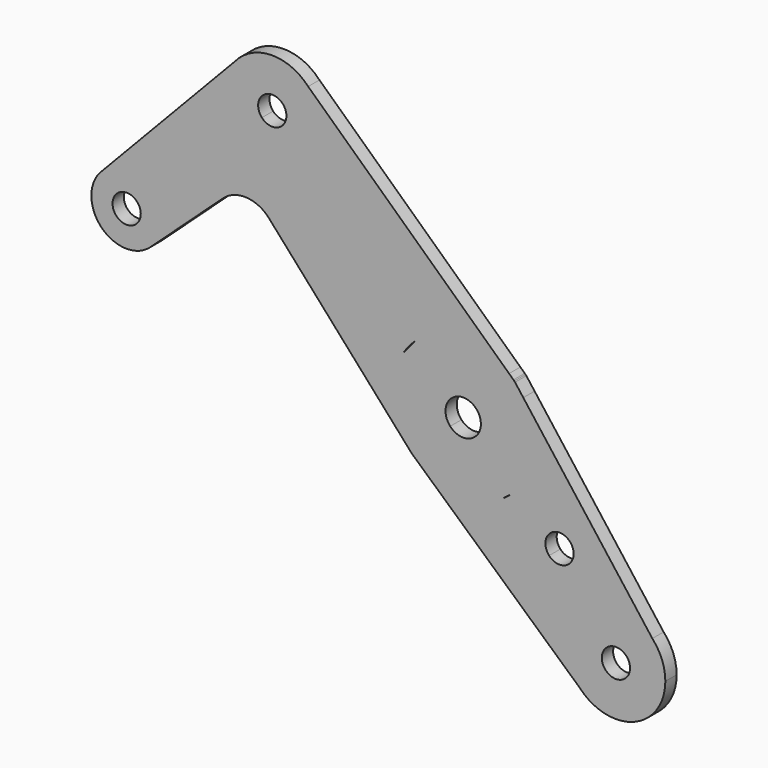
from build123d import *

# Parameters (mm, degrees)
F1_DEPTH = 3.175


with BuildPart() as f1:
    # F0 (on Front) → F1 (new body)
    with BuildSketch(Plane.XZ):
        with BuildLine():
            ThreePointArc((-2.6877932952, 2.9286835289), (1.5995582019, 3.6390704265), (3.9751, 0))
            ThreePointArc((3.9751, 0), (3.6390704265, -1.5995582019), (2.6877932952, -2.9286835289))
            Line((2.6877932952, -2.9286835289), (10.7339987827, -11.6960204828))
            ThreePointArc((10.7339987827, -11.6960204828), (14.5330288597, -6.3880119883), (15.875, 0))
            ThreePointArc((15.875, 0), (15.2734304328, 4.3287351287), (13.5143136611, 8.3294028158))
            Line((13.5143136611, 8.3294028158), (11.6590601378, 10.7741329908))
            Line((11.6590601378, 10.7741329908), (11.4851871667, 10.9592928944))
            Line((11.4851871667, 10.9592928944), (11.3083739877, 11.1416472191))
            Line((11.3083739877, 11.1416472191), (10.3225973322, 12.0606637179))
            ThreePointArc((10.3225973322, 12.0606637179), (-0.2748708071, 15.8726201693), (-10.7339987827, 11.6960204828))
            Line((-10.7339987827, 11.6960204828), (-2.6877932952, 2.9286835289))
        make_face()
        with BuildLine():
            ThreePointArc((-2.9286835289, -2.6877932952), (-3.9714488487, 0.1703351178), (-2.6877932952, 2.9286835289))
            Line((-2.6877932952, 2.9286835289), (-10.7339987827, 11.6960204828))
            Line((-10.7339987827, 11.6960204828), (-13.3268527784, 8.6261590538))
            ThreePointArc((-13.3268527784, 8.6261590538), (-15.8291292061, -1.2059409505), (-11.8662618768, -10.5454944915))
            Line((-11.8662618768, -10.5454944915), (-11.6960204828, -10.7339987827))
            Line((-11.6960204828, -10.7339987827), (-2.9286835289, -2.6877932952))
        make_face()
        with BuildLine():
            Line((10.7339987827, -11.6960204828), (2.6877932952, -2.9286835289))
            ThreePointArc((2.6877932952, -2.9286835289), (-0.1703351178, -3.9714488487), (-2.9286835289, -2.6877932952))
            Line((-2.9286835289, -2.6877932952), (-11.6960204828, -10.7339987827))
            Line((-11.6960204828, -10.7339987827), (-11.5227849075, -10.9197551701))
            Line((-11.5227849075, -10.9197551701), (-9.6887004006, -12.5755600093))
            ThreePointArc((-9.6887004006, -12.5755600093), (-0.5030588817, -15.8670273448), (8.8726348179, -13.1640410357))
            Line((8.8726348179, -13.1640410357), (10.7339987827, -11.6960204828))
        make_face()
        with BuildLine():
            Line((-35.5304524208, 38.714826384), (-10.7339987827, 11.6960204828))
            ThreePointArc((-10.7339987827, 11.6960204828), (-0.2748708071, 15.8726201693), (10.3225973322, 12.0606637179))
            Line((10.3225973322, 12.0606637179), (-34.8667395835, 54.189624641))
            ThreePointArc((-34.8667395835, 54.189624641), (-32.7298053677, 50.7575739011), (-31.9836005106, 46.7840819312))
            ThreePointArc((-31.9836005106, 46.7840819312), (-32.9094460222, 42.3768990566), (-35.5304524208, 38.714826384))
        make_face()
        with BuildLine():
            ThreePointArc((-13.3268527784, 8.6261590538), (-12.1279494046, 10.2434597788), (-10.7339987827, 11.6960204828))
            Line((-10.7339987827, 11.6960204828), (-35.5304524208, 38.714826384))
            ThreePointArc((-35.5304524208, 38.714826384), (-43.4053109787, 35.8417471462), (-51.0052506778, 39.3785392213))
            Line((-51.0052506778, 39.3785392213), (-69.8368422411, 22.0958847311))
            ThreePointArc((-69.8368422411, 22.0958847311), (-68.2881475559, 19.6085836711), (-67.7473524824, 16.7288853397))
            ThreePointArc((-67.7473524824, 16.7288853397), (-68.4183380526, 13.5348793456), (-70.3178530911, 10.8808750983))
            Line((-70.3178530911, 10.8808750983), (-54.0081981098, 25.8490274689))
            ThreePointArc((-54.0081981098, 25.8490274689), (-48.7323738618, 27.7047005709), (-43.6967288942, 25.2715700939))
            Line((-43.6967288942, 25.2715700939), (-20.9173687453, -0.3607843802))
            Line((-20.9173687453, -0.3607843802), (-13.3268527784, 8.6261590538))
        make_face()
        with BuildLine():
            Line((19.3211978133, -21.0528368739), (10.7339987827, -11.6960204828))
            ThreePointArc((10.7339987827, -11.6960204828), (9.830757416, -12.4648238507), (8.8726348179, -13.1640410357))
            Line((8.8726348179, -13.1640410357), (-0.6862483149, -20.7029410933))
            Line((-0.6862483149, -20.7029410933), (26.1615817665, -44.9410646928))
            ThreePointArc((26.1615817665, -44.9410646928), (23.2465029972, -36.9510890975), (26.8349969566, -29.240051207))
            Line((26.8349969566, -29.240051207), (19.3211978133, -21.0528368739))
        make_face()
        with BuildLine():
            ThreePointArc((15.875, 0), (14.5330288597, -6.3880119883), (10.7339987827, -11.6960204828))
            Line((10.7339987827, -11.6960204828), (19.3211978133, -21.0528368739))
            Line((19.3211978133, -21.0528368739), (26.8349969566, -29.240051207))
            ThreePointArc((26.8349969566, -29.240051207), (34.824972552, -26.3249724376), (42.5360104425, -29.9134663971))
            Line((42.5360104425, -29.9134663971), (13.5143136611, 8.3294028158))
            ThreePointArc((13.5143136611, 8.3294028158), (15.2734304328, 4.3287351287), (15.875, 0))
        make_face()
        with BuildLine():
            ThreePointArc((24.8354019053, -18.9060371125), (22.812281241, -21.8647190819), (19.3211978133, -21.0528368739))
            ThreePointArc((19.3211978133, -21.0528368739), (20.5085225697, -15.9473551431), (24.8354019053, -18.9060371125))
        make_face(mode=Mode.SUBTRACT)
        with BuildLine():
            ThreePointArc((-11.8662618768, -10.5454944915), (-15.8291292061, -1.2059409505), (-13.3268527784, 8.6261590538))
            Line((-13.3268527784, 8.6261590538), (-20.9173687453, -0.3607843802))
            Line((-20.9173687453, -0.3607843802), (-11.8662618768, -10.5454944915))
        make_face()
        with BuildLine():
            ThreePointArc((-51.0052506778, 39.3785392213), (-43.4053109787, 35.8417471462), (-35.5304524208, 38.714826384))
            Line((-35.5304524208, 38.714826384), (-40.7891953741, 44.4448778346))
            ThreePointArc((-40.7891953741, 44.4448778346), (-43.0720455442, 43.6119981862), (-45.2751992272, 44.6372821746))
            Line((-45.2751992272, 44.6372821746), (-51.0052506778, 39.3785392213))
        make_face()
        with BuildLine():
            Line((-40.7891953741, 44.4448778346), (-35.5304524208, 38.714826384))
            ThreePointArc((-35.5304524208, 38.714826384), (-32.9094460222, 42.3768990566), (-31.9836005106, 46.7840819312))
            ThreePointArc((-31.9836005106, 46.7840819312), (-32.7298053677, 50.7575739011), (-34.8667395835, 54.189624641))
            ThreePointArc((-34.8667395835, 54.189624641), (-42.4666792826, 57.7264167162), (-50.3415378405, 54.8533374783))
            Line((-50.3415378405, 54.8533374783), (-51.3633206037, 53.7794470598))
            ThreePointArc((-51.3633206037, 53.7794470598), (-53.8850057244, 46.5118413574), (-51.0052506778, 39.3785392213))
            Line((-51.0052506778, 39.3785392213), (-45.2751992272, 44.6372821746))
            ThreePointArc((-45.2751992272, 44.6372821746), (-44.0878744632, 49.7427639018), (-39.7609951306, 46.7840819312))
            ThreePointArc((-39.7609951306, 46.7840819312), (-40.0293893587, 45.5064795335), (-40.7891953741, 44.4448778346))
        make_face()
        with BuildLine():
            Line((-0.6862483149, -20.7029410933), (8.8726348179, -13.1640410357))
            ThreePointArc((8.8726348179, -13.1640410357), (-0.5030588817, -15.8670273448), (-9.6887004006, -12.5755600093))
            Line((-9.6887004006, -12.5755600093), (-0.6862483149, -20.7029410933))
        make_face()
        with BuildLine():
            Line((-69.8368422411, 22.0958847311), (-51.0052506778, 39.3785392213))
            ThreePointArc((-51.0052506778, 39.3785392213), (-53.8850057244, 46.5118413574), (-51.3633206037, 53.7794470598))
            Line((-51.3633206037, 53.7794470598), (-81.0518518738, 22.5768955811))
            ThreePointArc((-81.0518518738, 22.5768955811), (-75.3447264485, 24.6590947021), (-69.8368422411, 22.0958847311))
        make_face()
        with BuildLine():
            ThreePointArc((42.5360104425, -29.9134663971), (34.824972552, -26.3249724376), (26.8349969566, -29.240051207))
            ThreePointArc((26.8349969566, -29.240051207), (23.2465029972, -36.9510890975), (26.1615817665, -44.9410646928))
            ThreePointArc((26.1615817665, -44.9410646928), (38.3803737684, -47.7826524421), (45.4612961045, -37.4272655449))
            ThreePointArc((45.4612961045, -37.4272655449), (44.7041830017, -33.3956878811), (42.5360104425, -29.9134663971))
        make_face()
        with BuildLine():
            ThreePointArc((37.5237961045, -37.4272655449), (33.0711937068, -40.3338713169), (32.201996348, -35.0880614484))
            ThreePointArc((32.201996348, -35.0880614484), (35.6263985022, -34.520659773), (37.5237961045, -37.4272655449))
        make_face(mode=Mode.SUBTRACT)
        with BuildLine():
            ThreePointArc((-67.7473524824, 16.7288853397), (-68.2881475559, 19.6085836711), (-69.8368422411, 22.0958847311))
            Line((-69.8368422411, 22.0958847311), (-73.3456483859, 18.8756850963))
            ThreePointArc((-73.3456483859, 18.8756850963), (-72.7261705118, 17.8807646723), (-72.5098524824, 16.7288853397))
            ThreePointArc((-72.5098524824, 16.7288853397), (-72.7782467105, 15.4512829421), (-73.5380527259, 14.3896812432))
            Line((-73.5380527259, 14.3896812432), (-70.3178530911, 10.8808750983))
            ThreePointArc((-70.3178530911, 10.8808750983), (-68.4183380526, 13.5348793456), (-67.7473524824, 16.7288853397))
        make_face()
        with BuildLine():
            Line((-73.3456483859, 18.8756850963), (-69.8368422411, 22.0958847311))
            ThreePointArc((-69.8368422411, 22.0958847311), (-75.3447264485, 24.6590947021), (-81.0518518738, 22.5768955811))
            ThreePointArc((-81.0518518738, 22.5768955811), (-81.5328627238, 11.3618859484), (-70.3178530911, 10.8808750983))
            Line((-70.3178530911, 10.8808750983), (-73.5380527259, 14.3896812432))
            ThreePointArc((-73.5380527259, 14.3896812432), (-78.8569362274, 16.8649357533), (-73.3456483859, 18.8756850963))
        make_face()
    extrude(amount=F1_DEPTH)


solid = f1.part
